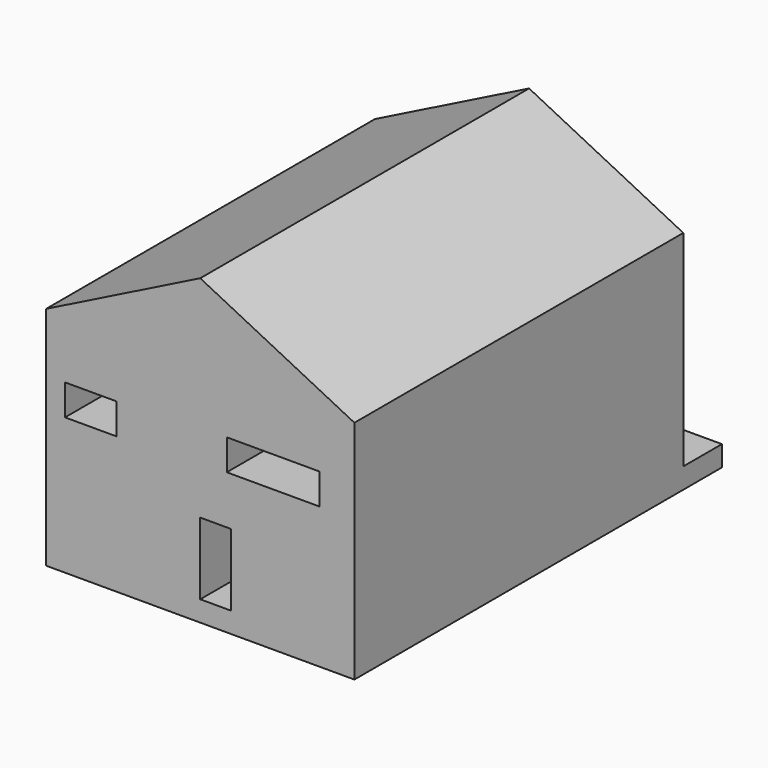
from build123d import *

# Parameters (mm, degrees)
F1_DEPTH     = 12192
F2_DEPTH     = 1432.56
F3_TEXT_SIZE = 781.6943857405
F4_DEPTH     = 518.16


# Not quite as in the source:
# - Text() gives the source's letters only with a copy of the font that has no kerning and outlines rounded to 1/6400 em; it was checked with that copy


with BuildPart() as f1:
    # F0 (on Front) → F1 (new body)
    with BuildSketch(Plane.XZ):
        Polygon((0, -6096), (0, 0), (-4572, 0), (-9144, 0), (-9144, -6096), (-4572, -6096), (-4572, -3962.4), (-3657.6, -3962.4), (-3657.6, -6096), align=None)
        Polygon((-8581.4990997314, -2193.4958192825), (-8581.4990997314, -1736.2958192825), (-7819.4990997314, -1736.2958192825), (-7057.4990997314, -1736.2958192825), (-7057.4990997314, -2193.4958192825), (-7057.4990997314, -2650.6958192825), (-7819.4990997314, -2650.6958192825), (-8581.4990997314, -2650.6958192825), align=None, mode=Mode.SUBTRACT)
        Polygon((-3785.2165699005, -2066.8612215042), (-3785.2165699005, -1609.6612215042), (-2413.6165699005, -1609.6612215042), (-1042.0165699005, -1609.6612215042), (-1042.0165699005, -2066.8612215042), (-1042.0165699005, -2524.0612215042), (-2413.6165699005, -2524.0612215042), (-3785.2165699005, -2524.0612215042), align=None, mode=Mode.SUBTRACT)
        Polygon((-4572, 0), (0, 0), (-4572, 2286), align=None)
        Polygon((-9144, 0), (-4572, 0), (-4572, 2286), align=None)
        Polygon((0, -6705.6), (0, -6096), (-3657.6, -6096), (-4572, -6096), (-9144, -6096), (-9144, -6705.6), align=None)
    extrude(amount=F1_DEPTH)

    # F0 (on Front) → F2 (join, symmetric)
    with BuildSketch(Plane.XZ):
        Polygon((0, -6705.6), (0, -6096), (-3657.6, -6096), (-4572, -6096), (-9144, -6096), (-9144, -6705.6), align=None)
    extrude(amount=F2_DEPTH, both=True)

    # F3 (on face) → F4 (join, symmetric)
    with BuildSketch(Plane.XY.offset(-6096)):
        with Locations((-7248.2886314392, 525.1343250275)):
            Text('CARTERS HOUSE', F3_TEXT_SIZE, font='Open Sans', font_style=FontStyle.BOLD, text_align=(TextAlign.LEFT, TextAlign.BOTTOM))
    extrude(amount=F4_DEPTH, both=True)


solid = f1.part
